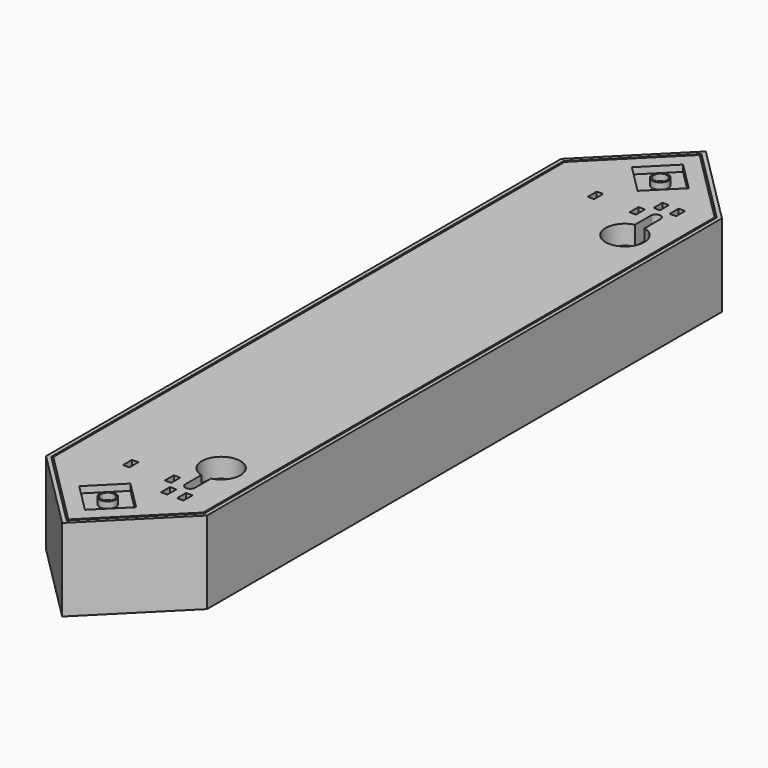
from build123d import *

# Parameters (mm, degrees)
F1_DEPTH       = 0.6
F2_DEPTH       = 25
F6_DEPTH       = 25
F7_R           = 2.2360679775
F8_DEPTH       = 1
F10_DEPTH      = 19
F10_TAPER      = 10
F11_R          = 2.525
F12_DEPTH      = 2
F13_R          = 2.125
F14_DEPTH      = 25.601
F14_DEPTH_BACK = 265
F15_SIZE       = 4
F16_W          = 11
F16_H          = 202
F17_DEPTH      = 1
F18_W          = 2
F18_H          = 3.5
F19_DEPTH      = 6.001


# Not quite as in the source:
# - an extrude ends at something that could not be found from the text; its depth is read off the source's solid
# - a pattern or mirror of a feature is missing from the dataset's text; its kind, count and spacing are read off the source's solid


with BuildPart() as f1:
    # F0 (on Top) → F1 (new body)
    with BuildSketch(Plane.XY):
        Polygon((25, 100), (0, 125), (-25, 100), (-25, -100), (0, -125), (25, -100), align=None)
        Polygon((23.8, 99.5029437252), (23.8, -99.5029437252), (0, -123.3029437252), (-23.8, -99.5029437252), (-23.8, 99.5029437252), (0, 123.3029437252), align=None, mode=Mode.SUBTRACT)
        Polygon((0, -123.3029437252), (23.8, -99.5029437252), (23.8, 99.5029437252), (0, 123.3029437252), (-23.8, 99.5029437252), (-23.8, -99.5029437252), align=None)
    extrude(amount=-F1_DEPTH)

    # F0 (on Top) → F2 (join)
    with BuildSketch(Plane.XY):
        Polygon((25, 100), (0, 125), (-25, 100), (-25, -100), (0, -125), (25, -100), align=None)
        Polygon((23.8, 99.5029437252), (23.8, -99.5029437252), (0, -123.3029437252), (-23.8, -99.5029437252), (-23.8, 99.5029437252), (0, 123.3029437252), align=None, mode=Mode.SUBTRACT)
    extrude(amount=F2_DEPTH)

    # F3 (on Front) → F4 (revolve)
    with BuildSketch(Plane.XZ):
        with BuildLine():
            Line((23.8, 17.527864045), (23.8, 19.7639320225))
            Line((23.8, 19.7639320225), (22.8, 19.7639320225))
            ThreePointArc((22.8, 19.7639320225), (23.0613872125, 18.5391871511), (23.8, 17.527864045))
        make_face()
    f4 = revolve(axis=Axis((23.3, 0, 19.7639320225), (-1, 0, 0)))

    # F4_copies: F4 across plane
    add(f4.mirror(Plane(origin=(0, 0, 0), x_dir=(0, 0, -1), z_dir=(-1, 0, 0))))


with BuildPart() as f6:
    # F5 (on face) → F6 (new body, through all)
    with BuildSketch(Plane.XY):
        Polygon((23.3, 99.295836944), (0, 122.595836944), (-23.3, 99.295836944), (-23.3, -99.295836944), (0, -122.595836944), (23.3, -99.295836944), align=None)
    extrude(amount=F6_DEPTH)

    # F7 (on face) → F8 (cut)
    with BuildSketch(Plane.YZ.offset(23.3)):
        with Locations((0, 19.7639320225)):
            Circle(F7_R)
    f8 = extrude(amount=-F8_DEPTH, mode=Mode.SUBTRACT)

    # F8_copies: F8 across plane
    add(f8.mirror(Plane(origin=(0, 0, 0), x_dir=(0, 0, -1), z_dir=(-1, 0, 0))), mode=Mode.SUBTRACT)

    # F9 (on face) → F10 (cut)
    with BuildSketch(Plane(origin=(0, 0, 0), x_dir=(1, 0, 0), z_dir=(0, 0, -1))):
        Polygon((0, -120.8987806691), (22.1, -98.7987806691), (22.1, 98.7987806691), (0, 120.8987806691), (-22.1, 98.7987806691), (-22.1, -98.7987806691), align=None)
    extrude(amount=-F10_DEPTH, taper=F10_TAPER, mode=Mode.SUBTRACT)

    # F11 (on face) → F12 (cut)
    with BuildSketch(Plane.XY.offset(25)):
        Polygon((8.8388347648, 107.3220297612), (0, 116.160864526), (-8.8388347648, 107.3220297612), (0, 98.4831949964), align=None)
        with Locations((0, 107.3220297612)):
            Circle(F11_R, mode=Mode.SUBTRACT)
        Polygon((-8.8388347648, -107.3220297612), (0, -116.160864526), (8.8388347648, -107.3220297612), (0, -98.4831949964), align=None)
        with Locations((0, -107.3220297612)):
            Circle(F11_R, mode=Mode.SUBTRACT)
    extrude(amount=-F12_DEPTH, mode=Mode.SUBTRACT)

    # F13 (on face) → F14 (cut, two sides)
    with BuildSketch(Plane.XY.offset(25)) as f14_sk:
        with Locations((0, -107.3220297612)):
            Circle(F13_R)
        with Locations((0, 107.3220297612)):
            Circle(F13_R)
    extrude(amount=-F14_DEPTH, mode=Mode.SUBTRACT)
    extrude(f14_sk.sketch, amount=F14_DEPTH_BACK, mode=Mode.SUBTRACT)

    # F15
    f15_edges = [f6.edges().sort_by_distance(p)[0] for p in [
        (-2.125, -107.32203, 19),
        (-2.125, 107.32203, 19),
    ]]
    chamfer(f15_edges, length=F15_SIZE)

    # F16 (on face) → F17 (cut)
    with BuildSketch(Plane(origin=(0, 0, 19), x_dir=(1, 0, 0), z_dir=(0, 0, -1))):
        Rectangle(F16_W, F16_H)
    extrude(amount=-F17_DEPTH, mode=Mode.SUBTRACT)

    # F18 (on face) → F19 (cut, through all)
    with BuildSketch(Plane(origin=(0, 0, 19), x_dir=(1, 0, 0), z_dir=(0, 0, -1))):
        with Locations((-6.5, -90.25)):
            Rectangle(F18_W, F18_H)
        with Locations((6.5, -90.25)):
            Rectangle(F18_W, F18_H)
        with Locations((-6.5, 90.25)):
            Rectangle(F18_W, F18_H)
        with Locations((6.5, 90.25)):
            Rectangle(F18_W, F18_H)
        with BuildLine():
            ThreePointArc((10.6248936833, 84.2205521788), (12.1248936833, 72.4110771595), (13.6248936833, 84.2205521788))
            Line((13.6248936833, 84.2205521788), (13.6248936833, 90.4110771595))
            ThreePointArc((13.6248936833, 90.4110771595), (12.1248936833, 91.9110771595), (10.6248936833, 90.4110771595))
            Line((10.6248936833, 90.4110771595), (10.6248936833, 84.2205521788))
        make_face()
        with Locations((9.6248936833, 95.6610771595)):
            Rectangle(F18_W, F18_H)
        with Locations((14.6248936833, 95.6610771595)):
            Rectangle(F18_W, F18_H)
        with BuildLine():
            Line((13.6248936833, -90.4110771595), (13.6248936833, -84.2205521788))
            ThreePointArc((13.6248936833, -84.2205521788), (12.1248936833, -72.4110771595), (10.6248936833, -84.2205521788))
            Line((10.6248936833, -84.2205521788), (10.6248936833, -90.4110771595))
            ThreePointArc((10.6248936833, -90.4110771595), (12.1248936833, -91.9110771595), (13.6248936833, -90.4110771595))
        make_face()
        with Locations((9.6248936833, -95.6610771595)):
            Rectangle(F18_W, F18_H)
        with Locations((14.6248936833, -95.6610771595)):
            Rectangle(F18_W, F18_H)
    extrude(amount=-F19_DEPTH, mode=Mode.SUBTRACT)


solid = Compound([f1.part, f6.part])
